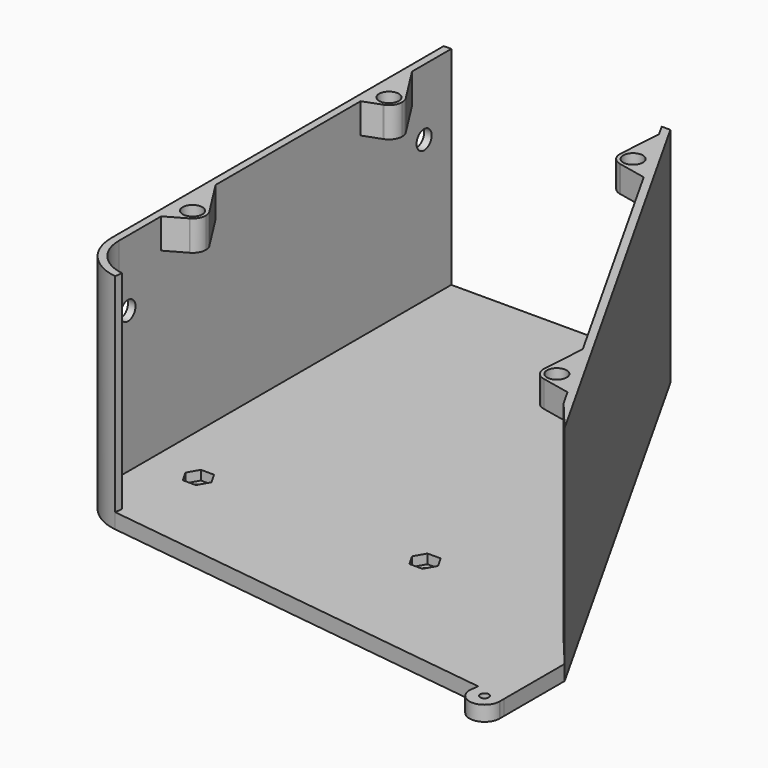
from build123d import *

# Parameters (mm, degrees)
F1_DEPTH  = 4
F3_DEPTH  = 55
F4_R      = 2.5
F5_DEPTH  = 2
F6_R      = 1.15
F7_DEPTH  = 2
F9_DEPTH  = 2.5
F10_R     = 1.7
F11_DEPTH = 1.5
F12_R     = 1.7
F13_DEPTH = 1.5
F15_DEPTH = 8
F17_DEPTH = 7
F18_R     = 2.6
F19_DEPTH = 6.5
F20_R     = 2.6
F21_DEPTH = 6.5
F22_W     = 110
F22_H     = 35
F23_DEPTH = 2.45


with BuildPart() as f1:
    # F0 (on Top) → F1 (new body)
    with BuildSketch(Plane.XY):
        with BuildLine():
            Line((-0.0348270737, 83.6430855933), (-60.0348270737, 83.6430855933))
            Line((-60.0348270737, 83.6430855933), (-60.0348270737, -26.3569144067))
            ThreePointArc((-60.0348270737, -26.3569144067), (-56.8036121084, -34.9342589227), (-48.7162364666, -39.2477197521))
            Line((-48.7162364666, -39.2477197521), (58.5887347718, -53.2440203484))
            Line((58.5887347718, -53.2440203484), (59.1074373156, -53.3116772019))
            ThreePointArc((59.1074373156, -53.3116772019), (62.8011202697, -51.776520456), (65.9774464875, -54.2077653548))
            Line((65.9774464875, -54.2077653548), (66.2837635334, -54.2477197521))
            Line((66.2837635334, -54.2477197521), (66.2837635334, -34.2477197521))
            Line((66.2837635334, -34.2477197521), (-0.0348270737, 83.6430855933))
        make_face()
        with BuildLine():
            Line((59.1074373156, -53.3116772019), (58.5887347718, -53.2440203484))
            Line((58.5887347718, -53.2440203484), (58.3714151196, -54.9101376817))
            ThreePointArc((58.3714151196, -54.9101376817), (58.6504322817, -54.0699295678), (59.1074373156, -53.3116772019))
        make_face()
        with BuildLine():
            Line((66.2835221478, -55.6989786465), (66.2837635334, -54.2477197521))
            Line((66.2837635334, -54.2477197521), (65.9774464875, -54.2077653548))
            ThreePointArc((65.9774464875, -54.2077653548), (66.2020782301, -54.9386771517), (66.2835221478, -55.6989786465))
        make_face()
        with BuildLine():
            Line((65.9774464875, -54.2077653548), (59.1074373156, -53.3116772019))
            ThreePointArc((59.1074373156, -53.3116772019), (58.6504322817, -54.0699295678), (58.3714151196, -54.9101376817))
            ThreePointArc((58.3714151196, -54.9101376817), (61.8425650137, -59.7185156245), (66.2835073084, -55.7881961))
            Line((66.2835073084, -55.7881961), (66.2835221478, -55.6989786465))
            ThreePointArc((66.2835221478, -55.6989786465), (66.2020782301, -54.9386771517), (65.9774464875, -54.2077653548))
        make_face()
        with BuildLine():
            ThreePointArc((66.2837635334, -55.7429221007), (66.2837031866, -55.7209500421), (66.2835221478, -55.6989786465))
            Line((66.2835221478, -55.6989786465), (66.2835073084, -55.7881961))
            ThreePointArc((66.2835073084, -55.7881961), (66.2836994767, -55.7655594629), (66.2837635334, -55.7429221007))
        make_face()
        with BuildLine():
            ThreePointArc((65.9774464875, -54.2077653548), (62.8011202697, -51.776520456), (59.1074373156, -53.3116772019))
            Line((59.1074373156, -53.3116772019), (65.9774464875, -54.2077653548))
        make_face()
    extrude(amount=F1_DEPTH)

    # F2 (on face) → F3 (join)
    with BuildSketch(Plane.XY.offset(4)):
        with BuildLine():
            ThreePointArc((-48.4575580984, -37.2645189297), (-55.300722103, -33.6146674587), (-58.0348270737, -26.3569144067))
            Line((-58.0348270737, -26.3569144067), (-58.0348270737, 83.6430855933))
            Line((-58.0348270737, 83.6430855933), (-60.0348270737, 83.6430855933))
            Line((-60.0348270737, 83.6430855933), (-60.0348270737, -26.3569144067))
            ThreePointArc((-60.0348270737, -26.3569144067), (-56.8036121084, -34.9342589227), (-48.7162364666, -39.2477197521))
            Line((-48.7162364666, -39.2477197521), (-48.4575580984, -37.2645189297))
        make_face()
        Polygon((-0.0348270737, 83.6430855933), (-2.3295637346, 83.6430855933), (59.1961841109, -25.7277544167), (66.2837635334, -34.2477197521), align=None)
    extrude(amount=F3_DEPTH)

    # F4 (on face) → F5 (cut, through all)
    with BuildSketch(Plane(origin=(-60.0348270737, 0, 0), x_dir=(0, -1, 0), z_dir=(-1, 0, 0))):
        with Locations((23.3569144067, 41.5)):
            Circle(F4_R)
        with Locations((-74.6430855933, 41.5)):
            Circle(F4_R)
    extrude(amount=-F5_DEPTH, mode=Mode.SUBTRACT)

    # F6 (on face) → F7 (cut)
    with BuildSketch(Plane.XY.offset(4)):
        with Locations((62.2837635334, -55.7429221007)):
            Circle(F6_R)
    extrude(amount=-F7_DEPTH, mode=Mode.SUBTRACT)

    # F8 (on face) → F9 (cut)
    with BuildSketch(Plane.XY.offset(4)):
        Polygon((-43.2614056757, -13.3569144067), (-46.7255072909, -13.3569144067), (-48.4575580984, -16.3569144067), (-46.7255072909, -19.3569144067), (-43.2614056757, -19.3569144067), (-41.5293548681, -16.3569144067), align=None)
        Polygon((16.7385943243, -13.3569144067), (13.2744927091, -13.3569144067), (11.5424419016, -16.3569144067), (13.2744927091, -19.3569144067), (16.7385943243, -19.3569144067), (18.4706451319, -16.3569144067), align=None)
    extrude(amount=-F9_DEPTH, mode=Mode.SUBTRACT)

    # F10 (on face) → F11 (cut, through all)
    with BuildSketch(Plane.XY.offset(1.5)):
        with Locations((15.0065435167, -16.3569144067)):
            Circle(F10_R)
    extrude(amount=-F11_DEPTH, mode=Mode.SUBTRACT)

    # F12 (on face) → F13 (cut, through all)
    with BuildSketch(Plane.XY.offset(1.5)):
        with Locations((-44.9934564833, -16.3569144067)):
            Circle(F12_R)
    extrude(amount=-F13_DEPTH, mode=Mode.SUBTRACT)

    # F14 (on face) → F15 (join)
    with BuildSketch(Plane.XY.offset(59)):
        with BuildLine():
            ThreePointArc((-52.7673478203, -9.3778442451), (-51.4986965275, -8.0981528472), (-51.0348270737, -6.3569144067))
            ThreePointArc((-51.0348270737, -6.3569144067), (-51.1491815724, -5.4695562268), (-51.4847725248, -4.6401828467))
            Line((-51.4847725248, -4.6401828467), (-51.6896180966, -4.3185852191))
            ThreePointArc((-51.6896180966, -4.3185852191), (-55.6052868974, -3.0246305403), (-58.0348270737, -6.3569143518))
            ThreePointArc((-58.0348270737, -6.3569143518), (-56.3204013937, -9.3671842197), (-52.856698827, -9.4283775088))
            Line((-52.856698827, -9.4283775088), (-52.7673478203, -9.3778442451))
        make_face()
        with BuildLine():
            Line((-51.6896180966, -4.3185852191), (-51.4847725248, -4.6401828467))
            ThreePointArc((-51.4847725248, -4.6401828467), (-51.5828126312, -4.4765924312), (-51.6896180966, -4.3185852191))
        make_face()
        with BuildLine():
            ThreePointArc((-58.0348270737, -6.3569143518), (-55.6052868974, -3.0246305403), (-51.6896180966, -4.3185852191))
            Line((-51.6896180966, -4.3185852191), (-58.0348270737, 5.6430855933))
            Line((-58.0348270737, 5.6430855933), (-58.0348270737, -6.3569143518))
        make_face()
        with BuildLine():
            Line((-58.0348270737, -12.3569144067), (-52.856698827, -9.4283775088))
            ThreePointArc((-52.856698827, -9.4283775088), (-56.3204013937, -9.3671842197), (-58.0348270737, -6.3569143518))
            Line((-58.0348270737, -6.3569143518), (-58.0348270737, -12.3569144067))
        make_face()
        with BuildLine():
            Line((-58.0348270737, 58.6430855933), (-58.0348270737, 53.6430855933))
            Line((-58.0348270737, 53.6430855933), (-53.4465181967, 55.3165883683))
            ThreePointArc((-53.4465181967, 55.3165883683), (-56.5892027611, 55.8094412023), (-58.0348270737, 58.6430855933))
        make_face()
        with BuildLine():
            Line((-53.2259221658, 55.3970467855), (-53.4465181967, 55.3165883683))
            ThreePointArc((-53.4465181967, 55.3165883683), (-53.3355452586, 55.3549671149), (-53.2259221658, 55.3970467855))
        make_face()
        with BuildLine():
            ThreePointArc((-58.0348270737, 58.6430855933), (-56.5892027611, 55.8094412023), (-53.4465181967, 55.3165883683))
            Line((-53.4465181967, 55.3165883683), (-53.2259221658, 55.3970467855))
            ThreePointArc((-53.2259221658, 55.3970467855), (-51.6338645457, 56.684918999), (-51.0348270737, 58.6430855933))
            ThreePointArc((-51.0348270737, 58.6430855933), (-51.1902368109, 59.6744516652), (-51.6426647732, 60.6142266912))
            ThreePointArc((-51.6426647732, 60.6142266912), (-55.5661931455, 61.9876758561), (-58.0348270737, 58.6430855933))
        make_face()
        with BuildLine():
            Line((-58.0348270737, 70.6430855933), (-58.0348270737, 58.6430855933))
            ThreePointArc((-58.0348270737, 58.6430855933), (-55.5661931455, 61.9876758561), (-51.6426647732, 60.6142266912))
            Line((-51.6426647732, 60.6142266912), (-58.0348270737, 70.6430855933))
        make_face()
    extrude(amount=-F15_DEPTH)

    # F16 (on face) → F17 (join)
    with BuildSketch(Plane.XY.offset(59)):
        with BuildLine():
            ThreePointArc((5.1432437589, 70.3590986219), (1.3150969821, 72.0555922251), (-1.3999848728, 68.86793967))
            ThreePointArc((-1.3999848728, 68.86793967), (-0.7360869019, 66.5821430027), (1.236164718, 65.2495326066))
            Line((1.236164718, 65.2495326066), (1.518343575, 65.1905478063))
            ThreePointArc((1.518343575, 65.1905478063), (4.3554664208, 65.9728286191), (5.5927848941, 68.6430855933))
            ThreePointArc((5.5927848941, 68.6430855933), (5.4785348868, 69.5300449986), (5.1432437589, 70.3590986219))
        make_face()
        with BuildLine():
            Line((-0.6419361775, 80.6430855933), (-1.3999848728, 68.86793967))
            ThreePointArc((-1.3999848728, 68.86793967), (1.3150969821, 72.0555922251), (5.1432437589, 70.3590986219))
            Line((5.1432437589, 70.3590986219), (-0.6419361775, 80.6430855933))
        make_face()
        with BuildLine():
            Line((8.9212866456, 63.6430855933), (5.1432437589, 70.3590986219))
            ThreePointArc((5.1432437589, 70.3590986219), (5.4785348868, 69.5300449986), (5.5927848941, 68.6430855933))
            ThreePointArc((5.5927848941, 68.6430855933), (4.3554664208, 65.9728286191), (1.518343575, 65.1905478063))
            Line((1.518343575, 65.1905478063), (8.9212866456, 63.6430855933))
        make_face()
        with BuildLine():
            Line((52.9593578497, -14.6409013336), (47.1741779383, -4.3569144067))
            Line((47.1741779383, -4.3569144067), (46.4675691299, -15.7187540374))
            ThreePointArc((46.4675691299, -15.7187540374), (49.3356306127, -12.9041816709), (52.9593578497, -14.6409013336))
        make_face()
        with BuildLine():
            ThreePointArc((52.9593578497, -14.6409013336), (49.3356306127, -12.9041816709), (46.4675691299, -15.7187540374))
            ThreePointArc((46.4675691299, -15.7187540374), (47.0023195828, -18.3067338942), (49.1940807829, -19.7831419097))
            ThreePointArc((49.1940807829, -19.7831419097), (52.1166281832, -19.0727811002), (53.4088990099, -16.3569144067))
            ThreePointArc((53.4088990099, -16.3569144067), (53.2946489962, -15.4699549767), (52.9593578497, -14.6409013336))
        make_face()
        with BuildLine():
            Line((56.7374007615, -21.3569144067), (52.9593578497, -14.6409013336))
            ThreePointArc((52.9593578497, -14.6409013336), (53.2946489962, -15.4699549767), (53.4088990099, -16.3569144067))
            ThreePointArc((53.4088990099, -16.3569144067), (52.1166281832, -19.0727811002), (49.1940807829, -19.7831419097))
            Line((49.1940807829, -19.7831419097), (56.7374007615, -21.3569144067))
        make_face()
    extrude(amount=-F17_DEPTH)

    # F18 (on face) → F19 (cut)
    with BuildSketch(Plane.XY.offset(59)):
        with Locations((-54.5348270737, -6.3569144067)):
            Circle(F18_R)
        with Locations((-54.5348270737, 58.6430855933)):
            Circle(F18_R)
    extrude(amount=-F19_DEPTH, mode=Mode.SUBTRACT)

    # F20 (on face) → F21 (cut)
    with BuildSketch(Plane.XY.offset(59)):
        with Locations((49.9088990099, -16.3569144067)):
            Circle(F20_R)
        with Locations((2.0927848941, 68.6430855933)):
            Circle(F20_R)
    extrude(amount=-F21_DEPTH, mode=Mode.SUBTRACT)

    # F22 (on face) → F23 (join)
    with BuildSketch(Plane(origin=(-60.0348270737, 0, 0), x_dir=(0, -1, 0), z_dir=(-1, 0, 0))):
        with Locations((-28.6430855933, 17.5)):
            Rectangle(F22_W, F22_H)
    extrude(amount=F23_DEPTH)


solid = f1.part
